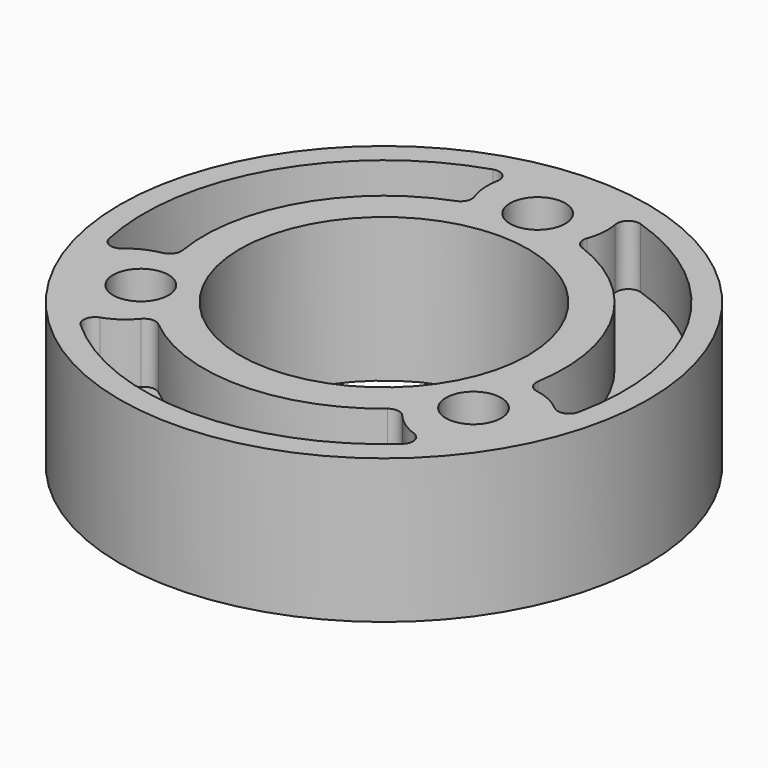
from build123d import *

# Parameters (mm, degrees)
F0_R            = 17.4625
F0_R_2          = 1.8288
F0_R_3          = 9.525
F1_DEPTH        = 9.525
F3_DEPTH        = 3.96875
F3_COPIES_COUNT = 3
F5_DEPTH        = 3.96875
F5_COPIES_COUNT = 3
F6_R            = 0.762


# Not quite as in the source:
# - a feature of the source that left no trace in its solid (it failed there, or was rolled back) is left out
# - a pattern or mirror of a feature is missing from the dataset's text; its kind, count and spacing are read off the source's solid


with BuildPart() as f1:
    # F0 (on Top) → F1 (new body)
    with BuildSketch(Plane.XY):
        Circle(F0_R)
        with Locations((-10.9985226281, -6.35)):
            Circle(F0_R_2, mode=Mode.SUBTRACT)
        with Locations((10.9985226281, -6.35)):
            Circle(F0_R_2, mode=Mode.SUBTRACT)
        Circle(F0_R_3, mode=Mode.SUBTRACT)
        with Locations((0, 12.7)):
            Circle(F0_R_2, mode=Mode.SUBTRACT)
    extrude(amount=F1_DEPTH)

    # F2 (on face) → F3 (cut)
    with BuildSketch(Plane.XY.offset(9.525)):
        with BuildLine():
            ThreePointArc((-3.3814051731, 11.4159926471), (-3.9685398143, 13.4529051128), (-3.4234536074, 15.5014705882))
            ThreePointArc((-3.4234536074, 15.5014705882), (-13.7481532851, 7.9375), (-15.1363941291, -4.7859375014))
            ThreePointArc((-15.1363941291, -4.7859375014), (-13.6348274895, -3.2895962613), (-11.5772422283, -2.7796135431))
            ThreePointArc((-11.5772422283, -2.7796135431), (-10.3111149638, 5.953125), (-3.3814051731, 11.4159926471))
        make_face()
    f3 = extrude(amount=-F3_DEPTH, mode=Mode.SUBTRACT)

    # F3_copies: F3 ×3 about axis
    f3_copies_axis = Axis((0, 0, 0), (0, 0, 1))
    for i in range(1, F3_COPIES_COUNT):
        add(f3.rotate(f3_copies_axis, i * 360 / F3_COPIES_COUNT), mode=Mode.SUBTRACT)

    # F4 (on face) → F5 (cut)
    with BuildSketch(Plane(origin=(0, 0, 0), x_dir=(1, 0, 0), z_dir=(0, 0, -1))):
        with BuildLine():
            ThreePointArc((-11.5772422283, 2.7796135431), (-13.6348274895, 3.2895962613), (-15.1363941291, 4.7859375014))
            ThreePointArc((-15.1363941291, 4.7859375014), (-13.7481532851, -7.9375), (-3.4234536074, -15.5014705882))
            ThreePointArc((-3.4234536074, -15.5014705882), (-3.9685398143, -13.4529051128), (-3.3814051731, -11.4159926471))
            ThreePointArc((-3.3814051731, -11.4159926471), (-10.3111149638, -5.953125), (-11.5772422283, 2.7796135431))
        make_face()
    f5 = extrude(amount=-F5_DEPTH, mode=Mode.SUBTRACT)

    # F5_copies: F5 ×3 about axis
    f5_copies_axis = Axis((0, 0, 0), (0, 0, 1))
    for i in range(1, F5_COPIES_COUNT):
        add(f5.rotate(f5_copies_axis, i * 360 / F5_COPIES_COUNT), mode=Mode.SUBTRACT)

    # F6
    f6_edges = [f1.edges().sort_by_distance(p)[0] for p in [
        (-15.136394, -4.785938, 7.540625),
        (-11.577242, -2.779614, 7.540625),
        (-3.381405, 11.415993, 7.540625),
        (-3.423454, 15.501471, 7.540625),
        (-3.381405, 11.415993, 1.984375),
        (-3.423454, 15.501471, 1.984375),
        (-11.577242, -2.779614, 1.984375),
        (-15.136394, -4.785938, 1.984375),
        (8.195837, -8.636379, 1.984375),
        (11.712941, -10.715533, 1.984375),
        (-8.195837, -8.636379, 1.984375),
        (-11.712941, -10.715533, 1.984375),
        (3.381405, 11.415993, 1.984375),
        (3.423454, 15.501471, 1.984375),
        (11.577242, -2.779614, 1.984375),
        (15.136394, -4.785938, 1.984375),
        (11.712941, -10.715533, 7.540625),
        (8.195837, -8.636379, 7.540625),
        (-11.712941, -10.715533, 7.540625),
        (-8.195837, -8.636379, 7.540625),
        (3.423454, 15.501471, 7.540625),
        (3.381405, 11.415993, 7.540625),
        (11.577242, -2.779614, 7.540625),
        (15.136394, -4.785938, 7.540625),
    ]]
    fillet(f6_edges, radius=F6_R)


solid = f1.part
